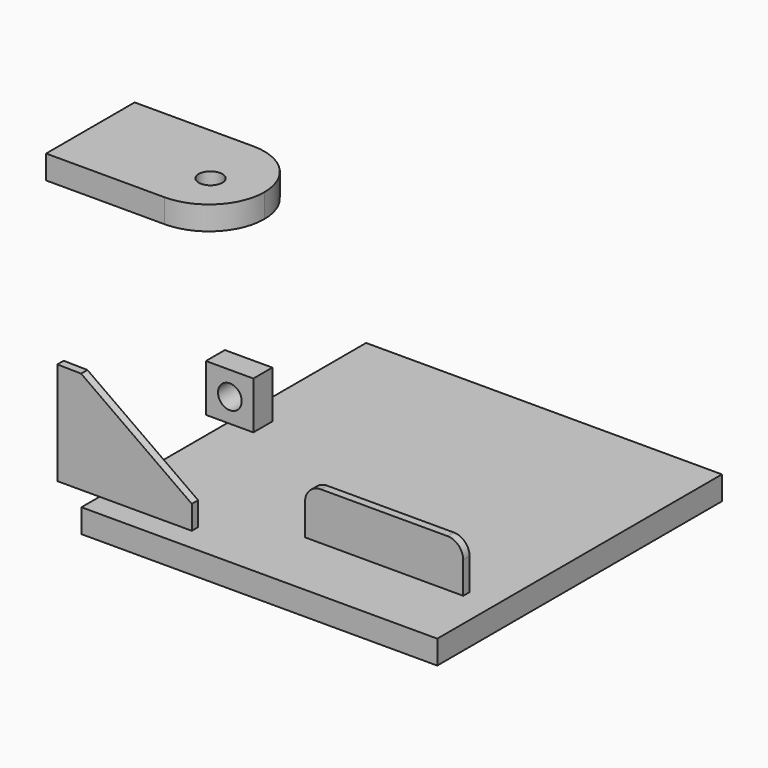
from build123d import *

# Parameters (mm, degrees)
F1_DEPTH = 6.35
F2_W     = 285.75
F2_H     = 19.05
F3_DEPTH = 285.75
F4_W     = 38.1
F4_H     = 38.1
F4_R     = 9.525
F5_DEPTH = 19.05
F6_W     = 139.7
F6_H     = 19.05
F7_DEPTH = 88.9
F8_R     = 9.525
F9_DEPTH = 76.2
F10_R    = 44.44999


# Not quite as in the source:
# - a fillet or chamfer is up to 0.001 mm smaller than in the source, because OpenCascade refuses the exact size


with BuildPart() as f1:
    # F0 (on Front) → F1 (new body)
    with BuildSketch(Plane.XZ):
        Polygon((-51.910363327, 45.5110752996), (-70.960363327, 45.8452826373), (-70.960363327, -36.7047173627), (36.989636673, -36.7047173627), (36.989636673, -17.6547173627), align=None)
    extrude(amount=F1_DEPTH)


with BuildPart() as f1b:
    # F0 (on Front) → F1, piece 2 (new body)
    with BuildSketch(Plane.XZ):
        with BuildLine():
            ThreePointArc((140.6862076044, 26.3294414565), (131.7059514833, 22.6096975776), (127.9862076044, 13.6294414565))
            Line((127.9862076044, 13.6294414565), (127.9862076044, -11.7705585435))
            Line((127.9862076044, -11.7705585435), (254.9862076044, -11.7705585435))
            Line((254.9862076044, -11.7705585435), (254.9862076044, 13.6294414565))
            ThreePointArc((254.9862076044, 13.6294414565), (251.2664637255, 22.6096975776), (242.2862076044, 26.3294414565))
            Line((242.2862076044, 26.3294414565), (140.6862076044, 26.3294414565))
        make_face()
    extrude(amount=F1_DEPTH)


with BuildPart() as f3:
    # F2 (on Front) → F3 (new body)
    with BuildSketch(Plane.XZ):
        with Locations((86.1693803481, -62.6063495874)):
            Rectangle(F2_W, F2_H)
    extrude(amount=-F3_DEPTH)


with BuildPart() as f5:
    # F4 (on Front) → F5 (new body)
    with BuildSketch(Plane.XZ):
        with Locations((62.2761137784, 63.7494698803)):
            Rectangle(F4_W, F4_H)
        with Locations((62.4856501818, 63.7494698803)):
            Circle(F4_R, mode=Mode.SUBTRACT)
    extrude(amount=-F5_DEPTH)


with BuildPart() as f7:
    # F6 (on Front) → F7 (new body)
    with BuildSketch(Plane.XZ):
        with Locations((-15.2637315914, 178.2262056568)):
            Rectangle(F6_W, F6_H)
    extrude(amount=-F7_DEPTH)

    # F8 (on face) → F9 (cut)
    with BuildSketch(Plane.XY.offset(187.7512056568)):
        with Locations((16.4862684086, 38.1)):
            Circle(F8_R)
    extrude(amount=-F9_DEPTH, mode=Mode.SUBTRACT)

    # F10 (radius 44.45 in the source; OpenCascade refuses exactly that, so slightly less here)
    f10_edges = [f7.edges().sort_by_distance(p)[0] for p in [
        (54.586268, 0, 178.226206),
        (54.586268, 88.9, 178.226206),
    ]]
    fillet(f10_edges, radius=F10_R)


solid = Compound([f1.part, f1b.part, f3.part, f5.part, f7.part])
